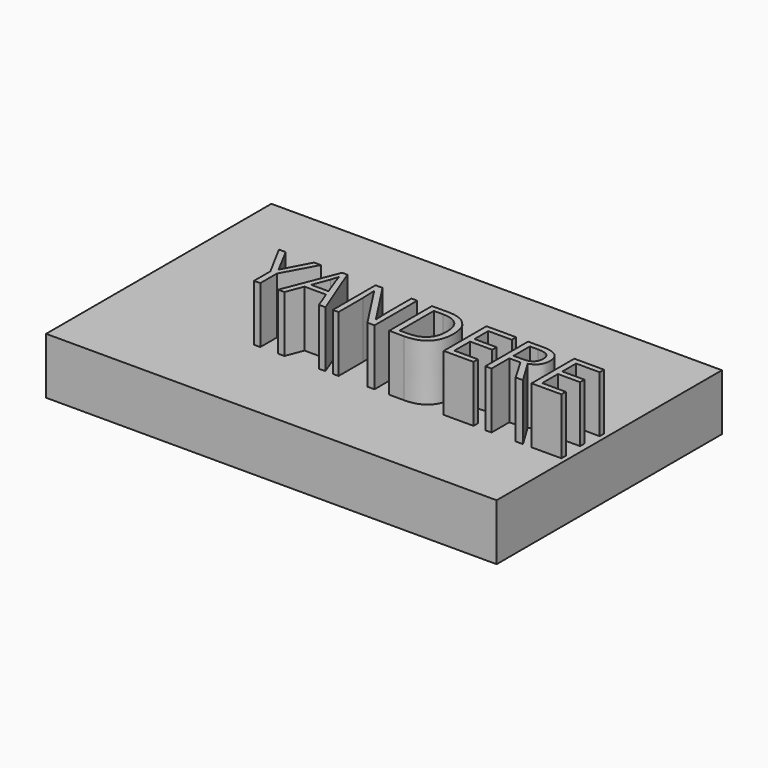
from build123d import *

# Parameters (mm, degrees)
F0_W         = 80
F0_H         = 50
F1_DEPTH     = 10
F2_TEXT_SIZE = 13.2828619563
F3_DEPTH     = 10


# Not quite as in the source:
# - Text() gives the source's letters only with a copy of the font that has no kerning and outlines rounded to 1/6400 em; it was checked with that copy


with BuildPart() as f1:
    # F0 (on Top) → F1 (new body)
    with BuildSketch(Plane.XY):
        Rectangle(F0_W, F0_H)
    extrude(amount=F1_DEPTH)

    # F2 (on face) → F3 (join)
    with BuildSketch(Plane.XY.offset(10)):
        with Locations((-18.5898739105, -9.5636606086)):
            Text('YANDERE', F2_TEXT_SIZE, font='Open Sans', text_align=(TextAlign.LEFT, TextAlign.BOTTOM))
    extrude(amount=F3_DEPTH)


solid = f1.part
